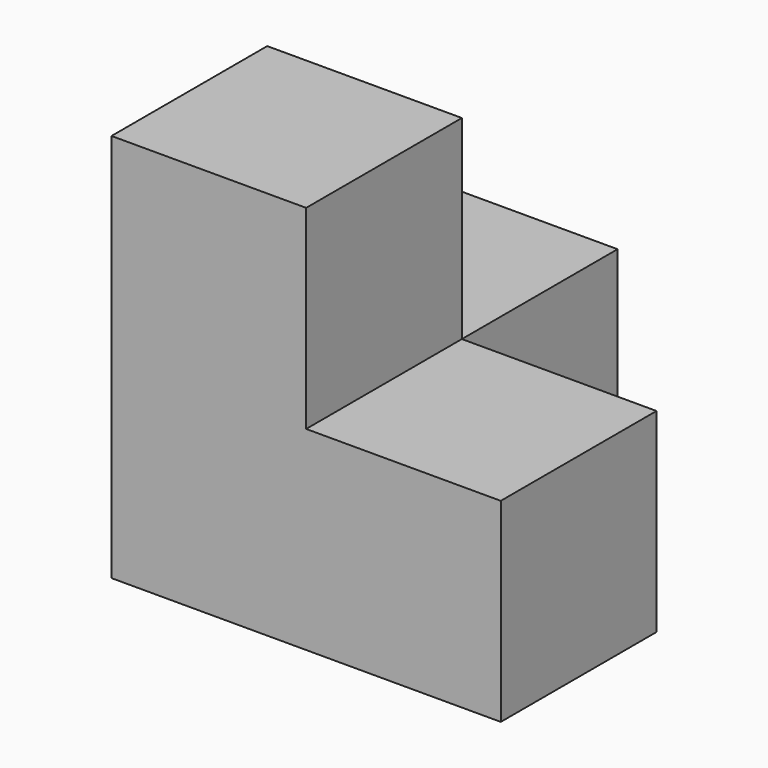
from build123d import *

# Parameters (mm, degrees)
F1_W     = 101.6
F1_H     = 101.6
F2_DEPTH = 50.8
F3_W     = 101.6
F3_H     = 101.6
F4_DEPTH = 101.6
F5_W     = 101.6
F5_H     = 101.6
F6_DEPTH = 101.6
F7_W     = 101.6
F7_H     = 101.6
F8_DEPTH = 101.6


# Not quite as in the source:
# - a variable given as a bare number and used for a length is read in inches; the dataset says mm whatever the document's units were


with BuildPart() as f2:
    # F1 (on Front) → F2 (new body, symmetric)
    with BuildSketch(Plane.XZ):
        Rectangle(F1_W, F1_H)
    extrude(amount=F2_DEPTH, both=True)

    # F3 (on face) → F4 (join)
    with BuildSketch(Plane.XZ.offset(50.8)):
        Rectangle(F3_W, F3_H)
    extrude(amount=F4_DEPTH)

    # F5 (on face) → F6 (join)
    with BuildSketch(Plane.YZ.offset(50.8)):
        with Locations((-101.6, 0)):
            Rectangle(F5_W, F5_H)
    extrude(amount=F6_DEPTH)

    # F7 (on face) → F8 (join)
    with BuildSketch(Plane.XY.offset(50.8)):
        with Locations((0, -101.6)):
            Rectangle(F7_W, F7_H)
    extrude(amount=F8_DEPTH)


solid = f2.part
